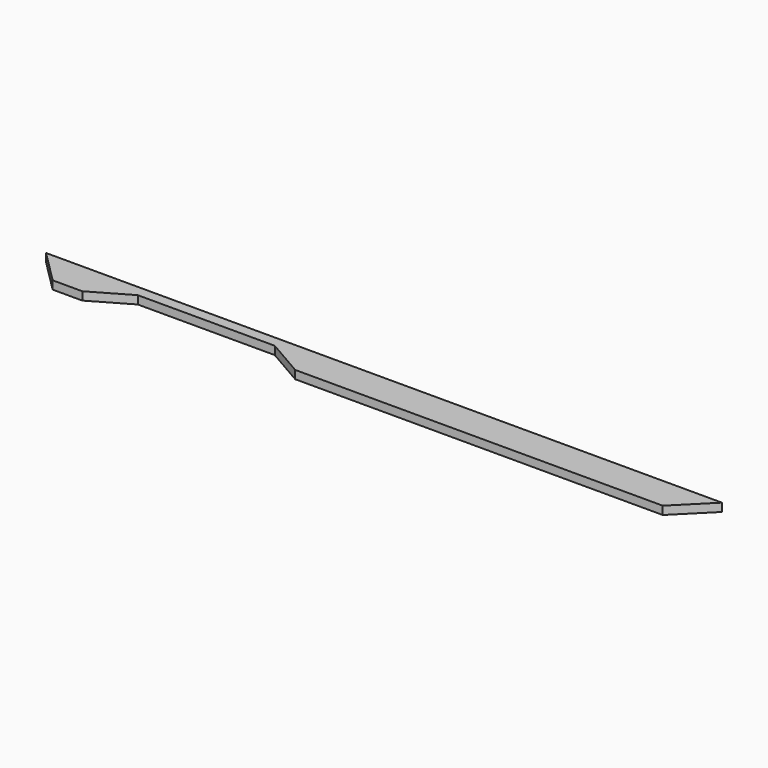
from build123d import *

# Parameters (mm, degrees)
F0_W     = 740
F0_H     = 36
F1_DEPTH = 9
F2_SIZE  = 35.99999
F4_DEPTH = 9


# Not quite as in the source:
# - a fillet or chamfer is up to 0.001 mm smaller than in the source, because OpenCascade refuses the exact size


with BuildPart() as f1:
    # F0 (on Top) → F1 (new body)
    with BuildSketch(Plane.XY):
        Rectangle(F0_W, F0_H)
    extrude(amount=F1_DEPTH)

    # F2 (size 36 in the source; OpenCascade refuses exactly that, so slightly less here)
    f2_edges = [f1.edges().sort_by_distance(p)[0] for p in [
        (-370, -18, 4.5),
        (370, -18, 4.5),
    ]]
    chamfer(f2_edges, length=F2_SIZE)

    # F3 (on face) → F4 (cut, through all)
    with BuildSketch(Plane.XY.offset(9)):
        Polygon((-301.5692193817, -18), (-68.4307806183, -18), (-110, 6), (-260, 6), align=None)
    extrude(amount=-F4_DEPTH, mode=Mode.SUBTRACT)


solid = f1.part
